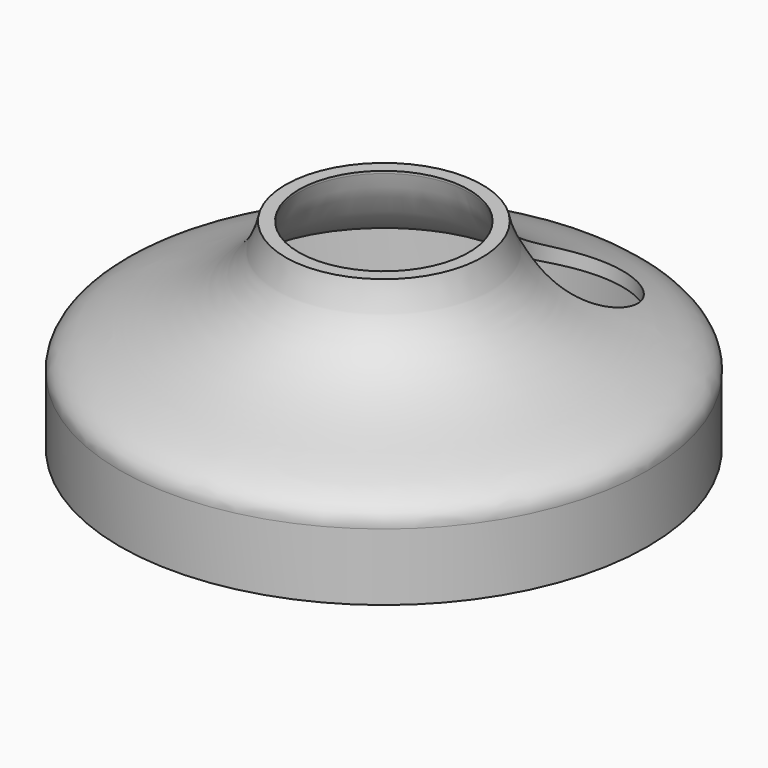
from build123d import *

# Parameters (mm, degrees)
F2_R          = 8
F3_DEPTH      = 25
F3_DEPTH_BACK = 25


# Not quite as in the source:
# - ends of sketch curves that miss each other by under 0.0002 mm in the source are joined
# - the dataset's text gives a spline's control points without its knots; the knots are read off the source's solid


with BuildPart() as f1:
    # F0 (on Front) → F1 (revolve)
    with BuildSketch(Plane.XZ):
        with BuildLine():
            Line((-37.45, -5), (-37.45, 0))
            Line((-37.45, 0), (-37.45, 4.9983821809))
            add(Edge.make_bspline(
                [(-37.45, 4.9983821809), (-37.4811403453, 5.5668856949), (-37.4141025822, 6.7150686136), (-35.1309255123, 7.3247914341)],
                knots=[0, 0, 0, 0, 3.2848571495, 3.2848571495, 3.2848571495, 3.2848571495], degree=3))
            add(Edge.make_bspline(
                [(-12.7335921145, 24.6349794144), (-12.9323365147, 23.5643204678), (-13.5111538376, 21.5523185481), (-14.8566836985, 18.9301540928), (-16.5850456529, 16.703993525), (-19.2632159702, 14.2268867189), (-23.0760434925, 11.9264351436), (-27.0305583413, 10.3150437437), (-30.0247840747, 9.2502993394), (-32.1169229262, 8.5244666288), (-33.8321158659, 7.8913152422), (-34.7652845833, 7.4947040144), (-35.1309255123, 7.3247914341)],
                knots=[0, 0, 0, 0, 0.0625, 0.125, 0.1875, 0.25, 0.375, 0.5, 0.5625, 0.625, 0.6875, 0.7349711774, 0.7349711774, 0.7349711774, 0.7349711774], degree=3))
            Line((-12.7335921145, 24.6349794144), (-12.7, 25))
            Line((-12.7, 25), (-14.7, 25))
            add(Edge.make_bspline(
                [(-14.7, 25), (-17.5202284008, 9.8071051762), (-40.336355567, 12.0357368141), (-39.45, 5)],
                knots=[0, 0, 0, 0, 31.820787231, 31.820787231, 31.820787231, 31.820787231], degree=3))
            Line((-39.45, 5), (-39.45, -5))
            Line((-39.45, -5), (-37.45, -5))
        make_face()
    revolve(axis=Axis((0, 0, 12.5), (0, 0, 1)))

    # F2 (on Top) → F3 (cut, two sides)
    with BuildSketch(Plane.XY) as f3_sk:
        with Locations((12, 20.7846096908)):
            Circle(F2_R)
    extrude(amount=F3_DEPTH, mode=Mode.SUBTRACT)
    extrude(f3_sk.sketch, amount=-F3_DEPTH_BACK, mode=Mode.SUBTRACT)


solid = f1.part
